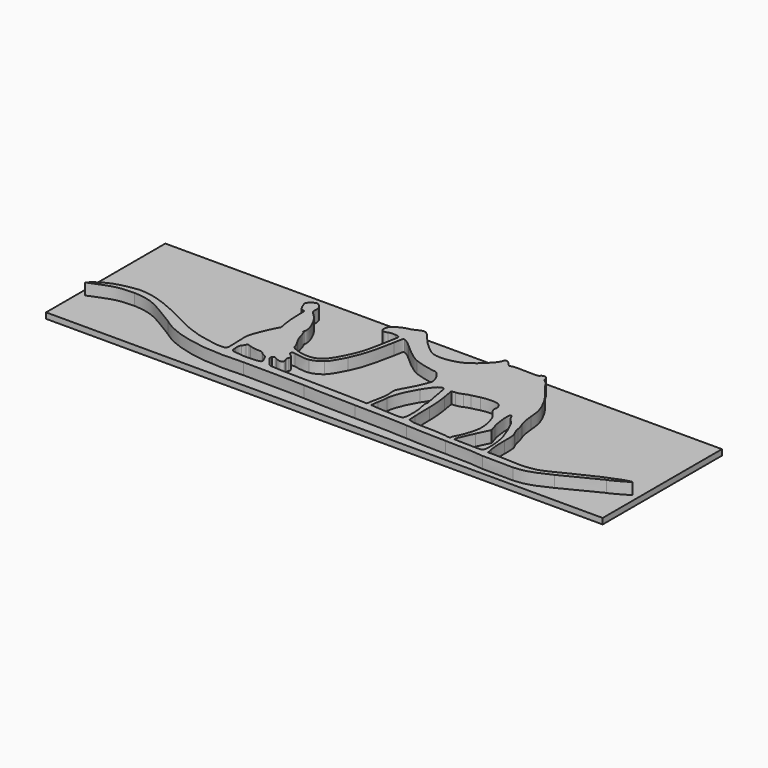
from build123d import *

# Parameters (mm, degrees)
F1_DEPTH = 2
F2_W     = 96.982617
F2_H     = 25.9708038449
F3_DEPTH = 1


# Not quite as in the source:
# - ends of sketch curves that miss each other by under 0.0002 mm in the source are joined


with BuildPart() as f1:
    # F0 (on Top) → F1 (new body)
    with BuildSketch(Plane.XY):
        with BuildLine():
            add(Edge.make_bspline(
                [(26.691874, -11.927583), (25.657716, -11.753169), (23.579804, -11.652992), (20.017703, -11.605818)],
                knots=[0, 0, 0, 0, 1, 1, 1, 1], degree=3))
            add(Edge.make_bspline(
                [(32.047701, -11.997616), (30.612274, -12.006111), (27.693789, -11.992423), (26.691874, -11.927583)],
                knots=[0, 0, 0, 0, 1, 1, 1, 1], degree=3))
            add(Edge.make_bspline(
                [(37.871114, -10.161981), (33.930318, -12.127275), (33.41182, -11.769755), (32.047701, -11.997616)],
                knots=[0, 0, 0, 0, 1, 1, 1, 1], degree=3))
            add(Edge.make_bspline(
                [(44.295003, -6.903307), (42.859271, -7.568347), (41.245168, -8.479321), (37.871114, -10.161981)],
                knots=[0, 0, 0, 0, 1, 1, 1, 1], degree=3))
            add(Edge.make_bspline(
                [(47.491308, -5.210222), (45.586999, -6.316471), (44.862402, -6.734321), (44.295003, -6.903307)],
                knots=[0, 0, 0, 0, 1, 1, 1, 1], degree=3))
            add(Edge.make_bspline(
                [(39.722405, -8.326128), (43.61465, -6.350352), (46.92664, -5.022), (47.491308, -5.210222)],
                knots=[0, 0, 0, 0, 1, 1, 1, 1], degree=3))
            add(Edge.make_bspline(
                [(34.083413, -10.674818), (35.419472, -10.469436), (35.868807, -10.282283), (39.722405, -8.326128)],
                knots=[0, 0, 0, 0, 1, 1, 1, 1], degree=3))
            add(Edge.make_bspline(
                [(30.829752, -10.767511), (32.09838, -10.859366), (33.061325, -10.831931), (34.083413, -10.674818)],
                knots=[0, 0, 0, 0, 1, 1, 1, 1], degree=3))
            add(Edge.make_bspline(
                [(27.835475, -10.636241), (28.491272, -10.636805), (29.838697, -10.695759), (30.829752, -10.767511)],
                knots=[0, 0, 0, 0, 1, 1, 1, 1], degree=3))
            Line((27.835475, -10.636241), (26.643115, -10.635394))
            Line((26.643115, -10.635394), (26.432574, -9.614794))
            add(Edge.make_bspline(
                [(26.243736, -6.546612), (26.231798, -7.672783), (26.316778, -9.053462), (26.432574, -9.614794)],
                knots=[0, 0, 0, 0, 1, 1, 1, 1], degree=3))
            add(Edge.make_bspline(
                [(25.941163, -3.965806), (26.21957, -4.42361), (26.262366, -4.788653), (26.243736, -6.546612)],
                knots=[0, 0, 0, 0, 1, 1, 1, 1], degree=3))
            add(Edge.make_bspline(
                [(25.506753, -2.676301), (25.567326, -3.092255), (25.762813, -3.672532), (25.941163, -3.965806)],
                knots=[0, 0, 0, 0, 1, 1, 1, 1], degree=3))
            add(Edge.make_bspline(
                [(25.086357, -1.303954), (25.257, -1.64279), (25.446176, -2.260348), (25.506753, -2.676301)],
                knots=[0, 0, 0, 0, 1, 1, 1, 1], degree=3))
            add(Edge.make_bspline(
                [(24.605044, 1.263363), (24.717103, -0.014918), (24.883104, -0.900359), (25.086357, -1.303954)],
                knots=[0, 0, 0, 0, 1, 1, 1, 1], degree=3))
            add(Edge.make_bspline(
                [(23.863274, 4.531575), (24.337653, 3.436908), (24.462861, 2.885252), (24.605044, 1.263363)],
                knots=[0, 0, 0, 0, 1, 1, 1, 1], degree=3))
            add(Edge.make_bspline(
                [(21.322066, 8.374536), (22.477729, 7.111947), (23.253369, 5.938978), (23.863274, 4.531575)],
                knots=[0, 0, 0, 0, 1, 1, 1, 1], degree=3))
            add(Edge.make_bspline(
                [(20.329696, 9.734855), (20.480886, 9.417804), (20.927454, 8.805659), (21.322066, 8.374536)],
                knots=[0, 0, 0, 0, 1, 1, 1, 1], degree=3))
            add(Edge.make_bspline(
                [(19.66083, 10.490819), (19.877514, 10.392089), (20.178502, 10.051907), (20.329696, 9.734855)],
                knots=[0, 0, 0, 0, 1, 1, 1, 1], degree=3))
            add(Edge.make_bspline(
                [(19.266859, 10.974237), (19.266859, 10.807083), (19.444145, 10.589546), (19.66083, 10.490819)],
                knots=[0, 0, 0, 0, 1, 1, 1, 1], degree=3))
            add(Edge.make_bspline(
                [(18.079443, 11.4049), (18.499601, 11.911161), (19.266859, 11.632887), (19.266859, 10.974237)],
                knots=[0, 0, 0, 0, 1, 1, 1, 1], degree=3))
            add(Edge.make_bspline(
                [(15.702776, 11.226798), (17.567461, 11.143867), (17.882389, 11.167466), (18.079443, 11.4049)],
                knots=[0, 0, 0, 0, 1, 1, 1, 1], degree=3))
            add(Edge.make_bspline(
                [(13.254905, 11.136069), (13.456338, 11.261867), (14.251544, 11.291339), (15.702776, 11.226798)],
                knots=[0, 0, 0, 0, 1, 1, 1, 1], degree=3))
            add(Edge.make_bspline(
                [(12.509505, 11.481029), (12.881336, 11.039134), (13.006749, 10.981095), (13.254905, 11.136069)],
                knots=[0, 0, 0, 0, 1, 1, 1, 1], degree=3))
            add(Edge.make_bspline(
                [(11.373995, 11.553462), (11.499087, 12.174475), (11.950222, 12.145696), (12.509505, 11.481029)],
                knots=[0, 0, 0, 0, 1, 1, 1, 1], degree=3))
            add(Edge.make_bspline(
                [(8.232086, 8.272724), (9.444577, 9.072652), (11.255092, 10.963166), (11.373995, 11.553462)],
                knots=[0, 0, 0, 0, 1, 1, 1, 1], degree=3))
            add(Edge.make_bspline(
                [(2.555208, 7.396924), (3.935566, 6.789079), (6.60823, 7.201406), (8.232086, 8.272724)],
                knots=[0, 0, 0, 0, 1, 1, 1, 1], degree=3))
            add(Edge.make_bspline(
                [(-1.028548, 10.636705), (0.141613, 9.188961), (1.714307, 7.767219), (2.555208, 7.396924)],
                knots=[0, 0, 0, 0, 1, 1, 1, 1], degree=3))
            add(Edge.make_bspline(
                [(-3.636776, 11.341174), (-2.305118, 12.035271), (-2.118141, 11.98477), (-1.028548, 10.636705)],
                knots=[0, 0, 0, 0, 1, 1, 1, 1], degree=3))
            add(Edge.make_bspline(
                [(-4.608944, 11.011186), (-4.422454, 11.011186), (-3.984979, 11.15968), (-3.636776, 11.341174)],
                knots=[0, 0, 0, 0, 1, 1, 1, 1], degree=3))
            add(Edge.make_bspline(
                [(-6.921202, 9.852124), (-6.75539, 10.169466), (-5.076213, 11.011186), (-4.608944, 11.011186)],
                knots=[0, 0, 0, 0, 1, 1, 1, 1], degree=3))
            add(Edge.make_bspline(
                [(-7.166509, 9.080484), (-7.10608, 9.362325), (-6.995691, 9.709565), (-6.921202, 9.852124)],
                knots=[0, 0, 0, 0, 1, 1, 1, 1], degree=3))
            add(Edge.make_bspline(
                [(-6.886714, 8.390501), (-7.214493, 8.539848), (-7.258931, 8.649432), (-7.166509, 9.080484)],
                knots=[0, 0, 0, 0, 1, 1, 1, 1], degree=3))
            add(Edge.make_bspline(
                [(-6.087449, 8.416014), (-6.386103, 8.267955), (-6.60259, 8.261043), (-6.886714, 8.390501)],
                knots=[0, 0, 0, 0, 1, 1, 1, 1], degree=3))
            add(Edge.make_bspline(
                [(-4.885298, 8.546917), (-5.325088, 8.586956), (-5.860167, 8.528686), (-6.087449, 8.416014)],
                knots=[0, 0, 0, 0, 1, 1, 1, 1], degree=3))
            add(Edge.make_bspline(
                [(-4.327069, 6.705908), (-3.962556, 8.444245), (-3.968378, 8.463444), (-4.885298, 8.546917)],
                knots=[0, 0, 0, 0, 1, 1, 1, 1], degree=3))
            add(Edge.make_bspline(
                [(-4.912555, 3.651953), (-4.690339, 4.7034), (-4.455945, 6.091288), (-4.327069, 6.705908)],
                knots=[0, 0, 0, 0, 1, 1, 1, 1], degree=3))
            add(Edge.make_bspline(
                [(-6.268639, -0.251482), (-5.481324, 1.374279), (-5.21201, 2.235045), (-4.912555, 3.651953)],
                knots=[0, 0, 0, 0, 1, 1, 1, 1], degree=3))
            add(Edge.make_bspline(
                [(-10.499816, -3.83024), (-8.533613, -3.850137), (-7.649067, -3.101972), (-6.268639, -0.251482)],
                knots=[0, 0, 0, 0, 1, 1, 1, 1], degree=3))
            add(Edge.make_bspline(
                [(-12.34829, -3.439656), (-11.799726, -3.649742), (-10.967913, -3.825505), (-10.499816, -3.83024)],
                knots=[0, 0, 0, 0, 1, 1, 1, 1], degree=3))
            add(Edge.make_bspline(
                [(-13.451093, -2.542252), (-13.360039, -2.987451), (-13.209782, -3.109721), (-12.34829, -3.439656)],
                knots=[0, 0, 0, 0, 1, 1, 1, 1], degree=3))
            add(Edge.make_bspline(
                [(-14.050104, -1.28163), (-13.778626, -1.691484), (-13.509073, -2.258765), (-13.451093, -2.542252)],
                knots=[0, 0, 0, 0, 1, 1, 1, 1], degree=3))
            add(Edge.make_bspline(
                [(-14.75295, 0.3986), (-14.637863, -0.115671), (-14.321582, -0.871773), (-14.050104, -1.28163)],
                knots=[0, 0, 0, 0, 1, 1, 1, 1], degree=3))
            add(Edge.make_bspline(
                [(-15.128334, 1.333633), (-15.036962, 1.333633), (-14.86804, 0.912868), (-14.75295, 0.3986)],
                knots=[0, 0, 0, 0, 1, 1, 1, 1], degree=3))
            add(Edge.make_bspline(
                [(-15.193482, 1.651808), (-15.249021, 1.476813), (-15.2197, 1.333633), (-15.128334, 1.333633)],
                knots=[0, 0, 0, 0, 1, 1, 1, 1], degree=3))
            add(Edge.make_bspline(
                [(-17.152237, 6.09825), (-15.989244, 5.026951), (-14.904089, 2.563609), (-15.193482, 1.651808)],
                knots=[0, 0, 0, 0, 1, 1, 1, 1], degree=3))
            add(Edge.make_bspline(
                [(-17.8911, 7.307744), (-17.963013, 6.931562), (-17.842225, 6.733837), (-17.152237, 6.09825)],
                knots=[0, 0, 0, 0, 1, 1, 1, 1], degree=3))
            add(Edge.make_bspline(
                [(-19.222681, 9.066898), (-18.522251, 9.314957), (-17.712019, 8.244556), (-17.8911, 7.307744)],
                knots=[0, 0, 0, 0, 1, 1, 1, 1], degree=3))
            add(Edge.make_bspline(
                [(-20.277608, 8.060329), (-20.277608, 8.321992), (-19.658782, 8.912449), (-19.222681, 9.066898)],
                knots=[0, 0, 0, 0, 1, 1, 1, 1], degree=3))
            add(Edge.make_bspline(
                [(-19.925522, 7.088288), (-20.119169, 7.500254), (-20.277608, 7.93767), (-20.277608, 8.060329)],
                knots=[0, 0, 0, 0, 1, 1, 1, 1], degree=3))
            add(Edge.make_bspline(
                [(-19.200448, 6.339262), (-19.478854, 6.339262), (-19.662722, 6.529203), (-19.925522, 7.088288)],
                knots=[0, 0, 0, 0, 1, 1, 1, 1], degree=3))
            add(Edge.make_bspline(
                [(-18.840967, 4.795859), (-18.827929, 6.286238), (-18.840403, 6.339262), (-19.200448, 6.339262)],
                knots=[0, 0, 0, 0, 1, 1, 1, 1], degree=3))
            add(Edge.make_bspline(
                [(-18.619956, 1.914238), (-18.748943, 2.650259), (-18.848395, 3.946988), (-18.840967, 4.795859)],
                knots=[0, 0, 0, 0, 1, 1, 1, 1], degree=3))
            Line((-18.619956, 1.914238), (-18.385435, 0.576019))
            Line((-18.385435, 0.576019), (-19.052072, -0.755429))
            add(Edge.make_bspline(
                [(-20.10558, -3.290454), (-19.892804, -2.628487), (-19.418724, -1.487728), (-19.052072, -0.755429)],
                knots=[0, 0, 0, 0, 1, 1, 1, 1], degree=3))
            add(Edge.make_bspline(
                [(-20.374295, -6.514081), (-20.482146, -4.67023), (-20.458704, -4.389043), (-20.10558, -3.290454)],
                knots=[0, 0, 0, 0, 1, 1, 1, 1], degree=3))
            add(Edge.make_bspline(
                [(-20.454158, -8.772733), (-20.310425, -8.599548), (-20.28853, -7.980327), (-20.374295, -6.514081)],
                knots=[0, 0, 0, 0, 1, 1, 1, 1], degree=3))
            add(Edge.make_bspline(
                [(-22.551261, -8.840043), (-22.189734, -8.932138), (-20.686305, -9.052455), (-20.454158, -8.772733)],
                knots=[0, 0, 0, 0, 1, 1, 1, 1], degree=3))
            add(Edge.make_bspline(
                [(-27.851372, -7.454809), (-25.010235, -8.592865), (-24.285655, -8.433511), (-22.551261, -8.840043)],
                knots=[0, 0, 0, 0, 1, 1, 1, 1], degree=3))
            add(Edge.make_bspline(
                [(-40.243704, -2.862128), (-35.903304, -2.819157), (-30.692511, -6.316754), (-27.851372, -7.454809)],
                knots=[0, 0, 0, 0, 1, 1, 1, 1], degree=3))
            add(Edge.make_bspline(
                [(-47.491309, -5.80712), (-45.485531, -3.773141), (-43.09291, -3.184699), (-40.243704, -2.862128)],
                knots=[0, 0, 0, 0, 1, 1, 1, 1], degree=3))
            add(Edge.make_bspline(
                [(-40.288849, -3.99858), (-43.5054, -4.014046), (-44.016327, -4.459926), (-47.491309, -5.80712)],
                knots=[0, 0, 0, 0, 1, 1, 1, 1], degree=3))
            add(Edge.make_bspline(
                [(-31.477007, -7.686528), (-35.436133, -5.43208), (-36.292785, -4.216749), (-40.288849, -3.99858)],
                knots=[0, 0, 0, 0, 1, 1, 1, 1], degree=3))
            add(Edge.make_bspline(
                [(-15.973183, -10.693086), (-24.157862, -11.196565), (-28.989867, -9.618706), (-31.477007, -7.686528)],
                knots=[0, 0, 0, 0, 1, 1, 1, 1], degree=3))
            add(Edge.make_bspline(
                [(-5.294509, -10.84232), (-6.276677, -10.750372), (-11.082388, -10.748692), (-15.973183, -10.693086)],
                knots=[0, 0, 0, 0, 1, 1, 1, 1], degree=3))
            add(Edge.make_bspline(
                [(3.832837, -11.100928), (-0.205035, -11.050642), (-4.312342, -10.934268), (-5.294509, -10.84232)],
                knots=[0, 0, 0, 0, 1, 1, 1, 1], degree=3))
            add(Edge.make_bspline(
                [(13.009823, -11.364837), (12.000356, -11.269974), (7.870711, -11.151215), (3.832837, -11.100928)],
                knots=[0, 0, 0, 0, 1, 1, 1, 1], degree=3))
            add(Edge.make_bspline(
                [(20.017703, -11.605818), (17.172838, -11.568142), (14.019292, -11.4597), (13.009823, -11.364837)],
                knots=[0, 0, 0, 0, 1, 1, 1, 1], degree=3))
        make_face()
        with BuildLine():
            add(Edge.make_bspline(
                [(-15.470111, -9.21405), (-14.129716, -9.144886), (-13.955574, -8.971759), (-14.29439, -8.342658)],
                knots=[0, 0, 0, 0, 1, 1, 1, 1], degree=3))
            add(Edge.make_bspline(
                [(-16.506109, -9.238135), (-16.315324, -9.221625), (-16.141181, -9.248661), (-15.470111, -9.21405)],
                knots=[0, 0, 0, 0, 1, 1, 1, 1], degree=3))
            add(Edge.make_bspline(
                [(-16.936207, -9.25535), (-16.760078, -9.263055), (-16.67816, -9.242932), (-16.506109, -9.238135)],
                knots=[0, 0, 0, 0, 1, 1, 1, 1], degree=3))
            add(Edge.make_bspline(
                [(-18.115007, -9.124591), (-17.668774, -9.162448), (-17.26376, -9.241025), (-16.936207, -9.25535)],
                knots=[0, 0, 0, 0, 1, 1, 1, 1], degree=3))
            add(Edge.make_bspline(
                [(-18.885155, -9.031692), (-18.62404, -9.101071), (-18.323882, -9.106867), (-18.115007, -9.124591)],
                knots=[0, 0, 0, 0, 1, 1, 1, 1], degree=3))
            add(Edge.make_bspline(
                [(-19.411485, -8.106494), (-19.365051, -8.825873), (-19.312566, -8.918128), (-18.885155, -9.031692)],
                knots=[0, 0, 0, 0, 1, 1, 1, 1], degree=3))
            add(Edge.make_bspline(
                [(-19.228281, -7.033118), (-19.378665, -7.208827), (-19.444522, -7.594681), (-19.411485, -8.106494)],
                knots=[0, 0, 0, 0, 1, 1, 1, 1], degree=3))
            add(Edge.make_bspline(
                [(-18.891821, -6.471696), (-18.94774, -6.629603), (-19.099147, -6.882242), (-19.228281, -7.033118)],
                knots=[0, 0, 0, 0, 1, 1, 1, 1], degree=3))
            add(Edge.make_bspline(
                [(-18.094636, -6.429984), (-18.73306, -6.204734), (-18.798493, -6.20816), (-18.891821, -6.471696)],
                knots=[0, 0, 0, 0, 1, 1, 1, 1], degree=3))
            add(Edge.make_bspline(
                [(-16.591704, -6.675371), (-17.035789, -6.675371), (-17.712107, -6.564945), (-18.094636, -6.429984)],
                knots=[0, 0, 0, 0, 1, 1, 1, 1], degree=3))
            add(Edge.make_bspline(
                [(-15.605687, -7.009081), (-15.746511, -6.745952), (-15.95505, -6.675371), (-16.591704, -6.675371)],
                knots=[0, 0, 0, 0, 1, 1, 1, 1], degree=3))
            add(Edge.make_bspline(
                [(-15.015829, -7.342789), (-15.246433, -7.274523), (-15.501251, -7.204224), (-15.605687, -7.009081)],
                knots=[0, 0, 0, 0, 1, 1, 1, 1], degree=3))
            add(Edge.make_bspline(
                [(-14.610188, -7.639371), (-14.750833, -7.46351), (-14.825786, -7.399048), (-15.015829, -7.342789)],
                knots=[0, 0, 0, 0, 1, 1, 1, 1], degree=3))
            add(Edge.make_bspline(
                [(-14.29439, -8.342658), (-14.347402, -8.213205), (-14.427347, -7.985333), (-14.610188, -7.639371)],
                knots=[0, 0, 0, 0, 1, 1, 1, 1], degree=3))
        make_face(mode=Mode.SUBTRACT)
        with BuildLine():
            add(Edge.make_bspline(
                [(0.742975, -9.573361), (1.147831, -9.604699), (1.578172, -9.579683), (2.697197, -9.621694)],
                knots=[0, 0, 0, 0, 1, 1, 1, 1], degree=3))
            add(Edge.make_bspline(
                [(-0.46479, -9.550958), (-0.084444, -9.579787), (0.250598, -9.553216), (0.742975, -9.573361)],
                knots=[0, 0, 0, 0, 1, 1, 1, 1], degree=3))
            add(Edge.make_bspline(
                [(-6.053492, -9.439582), (-3.015895, -9.480741), (-0.691538, -9.520616), (-0.46479, -9.550958)],
                knots=[0, 0, 0, 0, 1, 1, 1, 1], degree=3))
            add(Edge.make_bspline(
                [(-12.161484, -9.254983), (-11.839686, -9.315353), (-9.09109, -9.39842), (-6.053492, -9.439582)],
                knots=[0, 0, 0, 0, 1, 1, 1, 1], degree=3))
            add(Edge.make_bspline(
                [(-13.207995, -8.452541), (-12.860368, -8.974384), (-12.602267, -9.172292), (-12.161484, -9.254983)],
                knots=[0, 0, 0, 0, 1, 1, 1, 1], degree=3))
            add(Edge.make_bspline(
                [(-13.903949, -7.532784), (-13.754273, -7.860176), (-13.473033, -8.102509), (-13.207995, -8.452541)],
                knots=[0, 0, 0, 0, 1, 1, 1, 1], degree=3))
            add(Edge.make_bspline(
                [(-13.887693, -7.05492), (-13.971099, -7.236778), (-13.952365, -7.394312), (-13.903949, -7.532784)],
                knots=[0, 0, 0, 0, 1, 1, 1, 1], degree=3))
            add(Edge.make_bspline(
                [(-13.118697, -7.056613), (-13.575251, -6.786922), (-13.619543, -6.786829), (-13.887693, -7.05492)],
                knots=[0, 0, 0, 0, 1, 1, 1, 1], degree=3))
            add(Edge.make_bspline(
                [(-11.933618, -6.510889), (-11.515531, -7.292094), (-12.192404, -7.603789), (-13.118697, -7.056613)],
                knots=[0, 0, 0, 0, 1, 1, 1, 1], degree=3))
            add(Edge.make_bspline(
                [(-11.936892, -5.926937), (-12.076465, -6.095113), (-12.075624, -6.24556), (-11.933618, -6.510889)],
                knots=[0, 0, 0, 0, 1, 1, 1, 1], degree=3))
            add(Edge.make_bspline(
                [(-12.467907, -4.949997), (-12.018445, -5.067534), (-11.703909, -5.646211), (-11.936892, -5.926937)],
                knots=[0, 0, 0, 0, 1, 1, 1, 1], degree=3))
            add(Edge.make_bspline(
                [(-12.087739, -4.31301), (-12.848404, -4.141148), (-12.682599, -4.70336), (-12.467907, -4.949997)],
                knots=[0, 0, 0, 0, 1, 1, 1, 1], degree=3))
            add(Edge.make_bspline(
                [(-9.484417, -4.538787), (-10.050733, -4.713415), (-11.796418, -4.359777), (-12.087739, -4.31301)],
                knots=[0, 0, 0, 0, 1, 1, 1, 1], degree=3))
            add(Edge.make_bspline(
                [(-7.506711, -3.570232), (-8.012919, -4.028056), (-8.867575, -4.458879), (-9.484417, -4.538787)],
                knots=[0, 0, 0, 0, 1, 1, 1, 1], degree=3))
            add(Edge.make_bspline(
                [(-5.693724, -0.728807), (-6.253808, -1.872106), (-7.061026, -3.254101), (-7.506711, -3.570232)],
                knots=[0, 0, 0, 0, 1, 1, 1, 1], degree=3))
            add(Edge.make_bspline(
                [(-3.571029, 6.60905), (-4.309653, 2.691746), (-4.809062, 1.077042), (-5.693724, -0.728807)],
                knots=[0, 0, 0, 0, 1, 1, 1, 1], degree=3))
            add(Edge.make_bspline(
                [(-3.054306, 8.226539), (-3.312776, 8.266933), (-3.27108, 8.19984), (-3.571029, 6.60905)],
                knots=[0, 0, 0, 0, 1, 1, 1, 1], degree=3))
            add(Edge.make_bspline(
                [(-1.499622, 7.20267), (-1.96536, 7.631659), (-2.647446, 8.162954), (-3.054306, 8.226539)],
                knots=[0, 0, 0, 0, 1, 1, 1, 1], degree=3))
            add(Edge.make_bspline(
                [(2.181261, 4.420303), (1.333084, 4.795698), (0.108982, 5.720992), (-1.499622, 7.20267)],
                knots=[0, 0, 0, 0, 1, 1, 1, 1], degree=3))
            add(Edge.make_bspline(
                [(6.000529, 3.50274), (5.330147, 3.50274), (2.977218, 4.068022), (2.181261, 4.420303)],
                knots=[0, 0, 0, 0, 1, 1, 1, 1], degree=3))
            add(Edge.make_bspline(
                [(7.491247, 1.806423), (7.159822, 2.674245), (6.431745, 3.50274), (6.000529, 3.50274)],
                knots=[0, 0, 0, 0, 1, 1, 1, 1], degree=3))
            add(Edge.make_bspline(
                [(7.443102, 0.069583), (7.763823, 1.018924), (7.765728, 1.087699), (7.491247, 1.806423)],
                knots=[0, 0, 0, 0, 1, 1, 1, 1], degree=3))
            add(Edge.make_bspline(
                [(6.408256, -2.170308), (6.793757, -1.482033), (7.259438, -0.474082), (7.443102, 0.069583)],
                knots=[0, 0, 0, 0, 1, 1, 1, 1], degree=3))
            add(Edge.make_bspline(
                [(5.32516, -5.239935), (5.206658, -4.291462), (5.183589, -4.356839), (6.408256, -2.170308)],
                knots=[0, 0, 0, 0, 1, 1, 1, 1], degree=3))
            add(Edge.make_bspline(
                [(5.187503, -7.272668), (5.343654, -6.54377), (5.394415, -5.794219), (5.32516, -5.239935)],
                knots=[0, 0, 0, 0, 1, 1, 1, 1], degree=3))
            add(Edge.make_bspline(
                [(4.835965, -9.062711), (4.893261, -8.713258), (5.051452, -7.907739), (5.187503, -7.272668)],
                knots=[0, 0, 0, 0, 1, 1, 1, 1], degree=3))
            Line((4.835965, -9.062711), (4.731788, -9.698078))
            Line((4.731788, -9.698078), (2.697197, -9.621694))
        make_face(mode=Mode.SUBTRACT)
        with BuildLine():
            add(Edge.make_bspline(
                [(11.251985, -9.689718), (11.507162, -9.212912), (11.466575, -6.48471), (11.194414, -5.819763)],
                knots=[0, 0, 0, 0, 1, 1, 1, 1], degree=3))
            add(Edge.make_bspline(
                [(10.04229, -9.986294), (10.912677, -10.008251), (11.107004, -9.960612), (11.251985, -9.689718)],
                knots=[0, 0, 0, 0, 1, 1, 1, 1], degree=3))
            add(Edge.make_bspline(
                [(5.522168, -9.668823), (5.599108, -9.748926), (8.38238, -9.94441), (10.04229, -9.986294)],
                knots=[0, 0, 0, 0, 1, 1, 1, 1], degree=3))
            add(Edge.make_bspline(
                [(5.678912, -8.427344), (5.553873, -9.06973), (5.483337, -9.628397), (5.522168, -9.668823)],
                knots=[0, 0, 0, 0, 1, 1, 1, 1], degree=3))
            add(Edge.make_bspline(
                [(5.912383, -6.703398), (5.909024, -7.00918), (5.803947, -7.784953), (5.678912, -8.427344)],
                knots=[0, 0, 0, 0, 1, 1, 1, 1], degree=3))
            add(Edge.make_bspline(
                [(7.807104, -1.945682), (6.754988, -3.641041), (5.923121, -5.729889), (5.912383, -6.703398)],
                knots=[0, 0, 0, 0, 1, 1, 1, 1], degree=3))
            add(Edge.make_bspline(
                [(9.934278, 0.332509), (9.406943, 0.332509), (8.852232, -0.261583), (7.807104, -1.945682)],
                knots=[0, 0, 0, 0, 1, 1, 1, 1], degree=3))
            add(Edge.make_bspline(
                [(10.678927, -2.086877), (10.337441, 0.21344), (10.300791, 0.332509), (9.934278, 0.332509)],
                knots=[0, 0, 0, 0, 1, 1, 1, 1], degree=3))
            add(Edge.make_bspline(
                [(11.081308, -4.229494), (11.049883, -4.064516), (10.828784, -3.096347), (10.678927, -2.086877)],
                knots=[0, 0, 0, 0, 1, 1, 1, 1], degree=3))
            add(Edge.make_bspline(
                [(11.040781, -4.675806), (11.123037, -4.402093), (11.112731, -4.394476), (11.081308, -4.229494)],
                knots=[0, 0, 0, 0, 1, 1, 1, 1], degree=3))
            add(Edge.make_bspline(
                [(11.194414, -5.819763), (10.976485, -4.838417), (11.019295, -4.747302), (11.040781, -4.675806)],
                knots=[0, 0, 0, 0, 1, 1, 1, 1], degree=3))
        make_face(mode=Mode.SUBTRACT)
        with BuildLine():
            add(Edge.make_bspline(
                [(25.679591, -10.26274), (25.941237, -9.292897), (25.76152, -7.175866), (25.286566, -5.632892)],
                knots=[0, 0, 0, 0, 1, 1, 1, 1], degree=3))
            add(Edge.make_bspline(
                [(24.221894, -10.598409), (25.447432, -10.596716), (25.598921, -10.561768), (25.679591, -10.26274)],
                knots=[0, 0, 0, 0, 1, 1, 1, 1], degree=3))
            add(Edge.make_bspline(
                [(21.711877, -10.548704), (22.340169, -10.577118), (23.469675, -10.599487), (24.221894, -10.598409)],
                knots=[0, 0, 0, 0, 1, 1, 1, 1], degree=3))
            Line((21.711877, -10.548704), (20.569526, -10.49704))
            Line((20.569526, -10.49704), (20.681086, -10.046182))
            add(Edge.make_bspline(
                [(21.850011, -7.392633), (21.268458, -8.604114), (20.742444, -9.798207), (20.681086, -10.046182)],
                knots=[0, 0, 0, 0, 1, 1, 1, 1], degree=3))
            Line((21.850011, -7.392633), (22.907376, -5.189948))
            Line((22.907376, -5.189948), (22.505379, -3.924051))
            add(Edge.make_bspline(
                [(22.262408, -0.168054), (21.933571, -0.168054), (22.092417, -2.623627), (22.505379, -3.924051)],
                knots=[0, 0, 0, 0, 1, 1, 1, 1], degree=3))
            add(Edge.make_bspline(
                [(22.701292, -0.757814), (22.54737, -0.433448), (22.349871, -0.168054), (22.262408, -0.168054)],
                knots=[0, 0, 0, 0, 1, 1, 1, 1], degree=3))
            add(Edge.make_bspline(
                [(23.294286, -1.515157), (23.122062, -1.422986), (22.855216, -1.082183), (22.701292, -0.757814)],
                knots=[0, 0, 0, 0, 1, 1, 1, 1], degree=3))
            add(Edge.make_bspline(
                [(25.286566, -5.632892), (24.712627, -3.768372), (23.737126, -1.752159), (23.294286, -1.515157)],
                knots=[0, 0, 0, 0, 1, 1, 1, 1], degree=3))
        make_face(mode=Mode.SUBTRACT)
        with BuildLine():
            add(Edge.make_bspline(
                [(19.905, -10.304452), (19.880842, -10.18974), (19.996451, -9.893017), (20.161893, -9.645068)],
                knots=[0, 0, 0, 0, 1, 1, 1, 1], degree=3))
            add(Edge.make_bspline(
                [(19.239802, -10.430343), (19.413549, -10.604093), (19.946831, -10.503165), (19.905, -10.304452)],
                knots=[0, 0, 0, 0, 1, 1, 1, 1], degree=3))
            add(Edge.make_bspline(
                [(14.624938, -10.190403), (16.289115, -10.180808), (19.138391, -10.328935), (19.239802, -10.430343)],
                knots=[0, 0, 0, 0, 1, 1, 1, 1], degree=3))
            add(Edge.make_bspline(
                [(12.845547, -10.013309), (13.152435, -10.114593), (13.953162, -10.194284), (14.624938, -10.190403)],
                knots=[0, 0, 0, 0, 1, 1, 1, 1], degree=3))
            Line((12.845547, -10.013309), (12.287565, -9.829159))
            Line((12.287565, -9.829159), (12.186496, -8.460833))
            add(Edge.make_bspline(
                [(12.108292, -5.257111), (12.095705, -6.26658), (12.130898, -7.708253), (12.186496, -8.460833)],
                knots=[0, 0, 0, 0, 1, 1, 1, 1], degree=3))
            add(Edge.make_bspline(
                [(11.804607, -1.586317), (12.014902, -2.768275), (12.123021, -4.075153), (12.108292, -5.257111)],
                knots=[0, 0, 0, 0, 1, 1, 1, 1], degree=3))
            add(Edge.make_bspline(
                [(11.493093, 0.272596), (11.484824, 0.25967), (11.625001, -0.576847), (11.804607, -1.586317)],
                knots=[0, 0, 0, 0, 1, 1, 1, 1], degree=3))
            add(Edge.make_bspline(
                [(12.179096, 0.371439), (11.810068, 0.330009), (11.501365, 0.285528), (11.493093, 0.272596)],
                knots=[0, 0, 0, 0, 1, 1, 1, 1], degree=3))
            add(Edge.make_bspline(
                [(13.263648, 0.669133), (13.036174, 0.546832), (12.548124, 0.412866), (12.179096, 0.371439)],
                knots=[0, 0, 0, 0, 1, 1, 1, 1], degree=3))
            add(Edge.make_bspline(
                [(14.344658, 1.036767), (13.977577, 0.956869), (13.491125, 0.791434), (13.263648, 0.669133)],
                knots=[0, 0, 0, 0, 1, 1, 1, 1], degree=3))
            add(Edge.make_bspline(
                [(15.679493, 1.35443), (15.312412, 1.259612), (14.711736, 1.116664), (14.344658, 1.036767)],
                knots=[0, 0, 0, 0, 1, 1, 1, 1], degree=3))
            add(Edge.make_bspline(
                [(18.699968, 1.410725), (18.119933, 1.641936), (16.689315, 1.615271), (15.679493, 1.35443)],
                knots=[0, 0, 0, 0, 1, 1, 1, 1], degree=3))
            add(Edge.make_bspline(
                [(19.33017, -0.07688), (19.539452, 0.468498), (19.229755, 1.199544), (18.699968, 1.410725)],
                knots=[0, 0, 0, 0, 1, 1, 1, 1], degree=3))
            add(Edge.make_bspline(
                [(20.390129, -1.858119), (19.683111, -1.086944), (19.232899, -0.330369), (19.33017, -0.07688)],
                knots=[0, 0, 0, 0, 1, 1, 1, 1], degree=3))
            add(Edge.make_bspline(
                [(21.370786, -5.896008), (21.497574, -4.654394), (20.972813, -2.493678), (20.390129, -1.858119)],
                knots=[0, 0, 0, 0, 1, 1, 1, 1], degree=3))
            add(Edge.make_bspline(
                [(20.161893, -9.645068), (20.623741, -8.952884), (21.260183, -6.979132), (21.370786, -5.896008)],
                knots=[0, 0, 0, 0, 1, 1, 1, 1], degree=3))
        make_face(mode=Mode.SUBTRACT)
    extrude(amount=F1_DEPTH)

    # F2 (on face) → F3 (join)
    with BuildSketch(Plane(origin=(0, 0, 0), x_dir=(1, 0, 0), z_dir=(0, 0, -1))):
        with Locations((-5e-07, 0.0122140776)):
            Rectangle(F2_W, F2_H)
    extrude(amount=F3_DEPTH)


solid = f1.part
